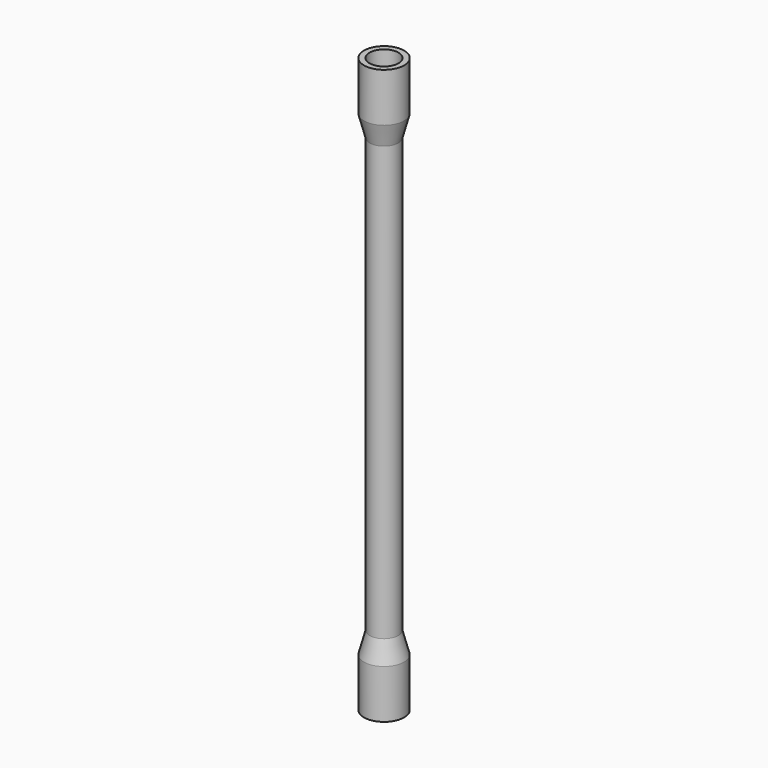
from build123d import *

# Parameters (mm, degrees)
F0_R         = 5
F1_DEPTH     = 75
F2_R         = 7
F2_R_2       = 5
F4_DEPTH     = 25
F3_R         = 7
F3_R_2       = 5
F5_DEPTH     = 25
F6_S5_R      = 5
F6_T6_DEPTH  = 12
F6_S11_R     = 5
F6_T12_DEPTH = 12
F7_R         = 5.05
F8_DEPTH     = 11
F9_R         = 5.05
F10_DEPTH    = 11


# Not quite as in the source:
# - a fillet or chamfer that OpenCascade refuses, or shapes differently, is made with other operations: its cross-section is extruded or revolved along the edge and cut away or added


with BuildPart() as f1:
    # F0 (on Top) → F1 (new body, symmetric)
    with BuildSketch(Plane.XY):
        Circle(F0_R)
    extrude(amount=F1_DEPTH, both=True)

    # F2 (on face) → F4 (join)
    with BuildSketch(Plane.XY.offset(75)):
        Circle(F2_R)
        Circle(F2_R_2, mode=Mode.SUBTRACT)
        Circle(F2_R_2)
    extrude(amount=F4_DEPTH)

    # F3 (on face) → F5 (join)
    with BuildSketch(Plane(origin=(0, 0, -75), x_dir=(1, 0, 0), z_dir=(0, 0, -1))):
        Circle(F3_R)
        Circle(F3_R_2, mode=Mode.SUBTRACT)
        Circle(F3_R_2)
    extrude(amount=F5_DEPTH)

    # F6: chamfer of 8 x 2.1435935394 on 2 edges, made by hand


with BuildPart() as f6_tool2:
    # F6_s3 → F6_t4 (revolve)
    with BuildSketch(Plane.XZ):
        Polygon((7, -83), (4.8564064606, -75), (7, -75), align=None)
    revolve(axis=Axis((0, 0, -75), (0, 0, -1)))

    # F6_s5 → F6_t6 (cut, symmetric)
    with BuildSketch(Plane.XY.offset(-79)):
        Circle(F6_S5_R)
    extrude(amount=F6_T6_DEPTH, both=True, mode=Mode.SUBTRACT)


with BuildPart() as f1_1:
    add(f1.part)

    # F6_t1: cut F6_tool2
    add(f6_tool2.part, mode=Mode.SUBTRACT)


with BuildPart() as f6_tool8:
    # F6_s9 → F6_t10 (revolve)
    with BuildSketch(Plane.XZ):
        Polygon((4.8564064606, 75), (7, 83), (7, 75), align=None)
    revolve(axis=Axis((0, 0, 75), (0, 0, 1)))

    # F6_s11 → F6_t12 (cut, symmetric)
    with BuildSketch(Plane.XY.offset(79)):
        Circle(F6_S11_R)
    extrude(amount=F6_T12_DEPTH, both=True, mode=Mode.SUBTRACT)


with BuildPart() as f1_2:
    add(f1_1.part)

    # F6_t7: cut F6_tool8
    add(f6_tool8.part, mode=Mode.SUBTRACT)

    # F7 (on face) → F8 (cut)
    with BuildSketch(Plane(origin=(0, 0, -100), x_dir=(1, 0, 0), z_dir=(0, 0, -1))):
        Circle(F7_R)
    extrude(amount=-F8_DEPTH, mode=Mode.SUBTRACT)

    # F9 (on face) → F10 (cut)
    with BuildSketch(Plane.XY.offset(100)):
        Circle(F9_R)
    extrude(amount=-F10_DEPTH, mode=Mode.SUBTRACT)


solid = f1_2.part
